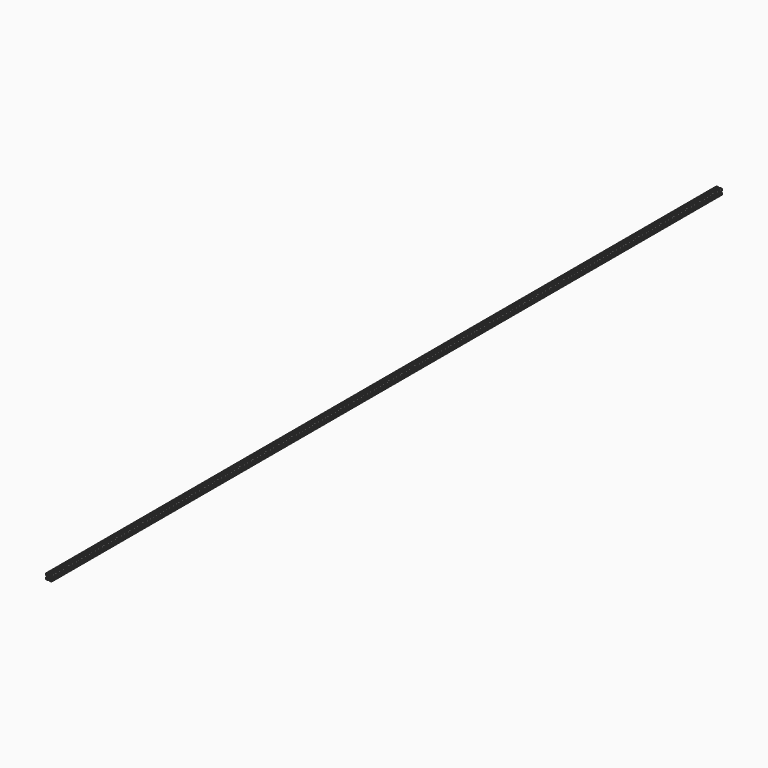
from build123d import *

# Parameters (mm, degrees)
F0_R     = 2.6035
F1_DEPTH = 1828.8


# Not quite as in the source:
# - ends of sketch curves that miss each other by under 0.0002 mm in the source are joined


with BuildPart() as f1:
    # F0 (on Front) → F1 (new body, symmetric)
    with BuildSketch(Plane.XZ):
        with BuildLine():
            ThreePointArc((-120.045226, 66.1162), (-119.5372260057, 65.6082762), (-120.0450736, 65.1002000229))
            ThreePointArc((-120.0450736, 65.1002000229), (-119.4277485161, 63.5840774839), (-117.9116260074, 62.9667530175))
            ThreePointArc((-117.9116260074, 62.9667530175), (-117.4035498, 63.4745999943), (-116.895626, 62.9666))
            Line((-116.895626, 62.9666), (-113.6783096, 62.9666))
            ThreePointArc((-113.6783096, 62.9666), (-113.1703096, 63.4746), (-112.6623096, 62.9666))
            Line((-112.6623096, 62.9666), (-111.688626, 62.9666))
            ThreePointArc((-111.688626, 62.9666), (-110.583726, 64.0715), (-111.688626, 65.1764))
            Line((-111.688626, 65.1764), (-113.8200162, 65.1764))
            ThreePointArc((-113.8200162, 65.1764), (-114.758677805, 65.8035936327), (-114.5384366897, 66.9108204897))
            Line((-114.5384366897, 66.9108204897), (-111.2083882, 70.2408552))
            ThreePointArc((-111.2083882, 70.2408552), (-110.1783528978, 70.9291175157), (-108.963333, 71.1708))
            Line((-108.963333, 71.1708), (-105.727119, 71.1708))
            ThreePointArc((-105.727119, 71.1708), (-104.5120991022, 70.9291175157), (-103.4820549697, 70.2408640303))
            Line((-103.4820549697, 70.2408640303), (-100.1520222, 66.9108136))
            ThreePointArc((-100.1520222, 66.9108136), (-99.931774195, 65.8035936327), (-100.8704358, 65.1764))
            Line((-100.8704358, 65.1764), (-103.001826, 65.1764))
            ThreePointArc((-103.001826, 65.1764), (-104.106726, 64.0715), (-103.001826, 62.9666))
            Line((-103.001826, 62.9666), (-102.0281424, 62.9666))
            ThreePointArc((-102.0281424, 62.9666), (-101.5201424, 63.4746), (-101.0121424, 62.9666))
            Line((-101.0121424, 62.9666), (-97.794826, 62.9666))
            ThreePointArc((-97.794826, 62.9666), (-97.2869022, 63.4745999943), (-96.7788260229, 62.9667524))
            ThreePointArc((-96.7788260229, 62.9667524), (-95.2627034839, 63.5840774839), (-94.6453790175, 65.1001999926))
            ThreePointArc((-94.6453790175, 65.1001999926), (-95.1532259943, 65.6082762), (-94.645226, 66.1162))
            Line((-94.645226, 66.1162), (-94.645226, 69.3335164))
            ThreePointArc((-94.645226, 69.3335164), (-95.153226, 69.8415164), (-94.645226, 70.3495164))
            Line((-94.645226, 70.3495164), (-94.645226, 71.3232))
            ThreePointArc((-94.645226, 71.3232), (-95.750126, 72.4281), (-96.855026, 71.3232))
            Line((-96.855026, 71.3232), (-96.855026, 69.1918098))
            ThreePointArc((-96.855026, 69.1918098), (-97.4822196327, 68.253148195), (-98.5894464897, 68.4733893103))
            Line((-98.5894464897, 68.4733893103), (-101.9194812, 71.8034378))
            ThreePointArc((-101.9194812, 71.8034378), (-102.6077435157, 72.8334731022), (-102.849426, 74.048493))
            Line((-102.849426, 74.048493), (-102.849426, 77.284707))
            ThreePointArc((-102.849426, 77.284707), (-102.6077435157, 78.4997268978), (-101.9194900303, 79.5297710303))
            Line((-101.9194900303, 79.5297710303), (-98.5894396, 82.8598038))
            ThreePointArc((-98.5894396, 82.8598038), (-97.4822196327, 83.080051805), (-96.855026, 82.1413902))
            Line((-96.855026, 82.1413902), (-96.855026, 80.01))
            ThreePointArc((-96.855026, 80.01), (-95.750126, 78.9051), (-94.645226, 80.01))
            Line((-94.645226, 80.01), (-94.645226, 80.9836836))
            ThreePointArc((-94.645226, 80.9836836), (-95.153226, 81.4916836), (-94.645226, 81.9996836))
            Line((-94.645226, 81.9996836), (-94.645226, 85.217))
            ThreePointArc((-94.645226, 85.217), (-95.1532259943, 85.7249238), (-94.6453784, 86.2329999771))
            ThreePointArc((-94.6453784, 86.2329999771), (-95.2627034839, 87.7491225161), (-96.7788259926, 88.3664469825))
            ThreePointArc((-96.7788259926, 88.3664469825), (-97.2869022, 87.8586000057), (-97.794826, 88.3666))
            Line((-97.794826, 88.3666), (-101.0121424, 88.3666))
            ThreePointArc((-101.0121424, 88.3666), (-101.5201424, 87.8586), (-102.0281424, 88.3666))
            Line((-102.0281424, 88.3666), (-103.001826, 88.3666))
            ThreePointArc((-103.001826, 88.3666), (-104.106726, 87.2617), (-103.001826, 86.1568))
            Line((-103.001826, 86.1568), (-100.8704358, 86.1568))
            ThreePointArc((-100.8704358, 86.1568), (-99.931774195, 85.5296063673), (-100.1520153103, 84.4223795103))
            Line((-100.1520153103, 84.4223795103), (-103.4820638, 81.0923448))
            ThreePointArc((-103.4820638, 81.0923448), (-104.5120991022, 80.4040824843), (-105.727119, 80.1624))
            Line((-105.727119, 80.1624), (-108.963333, 80.1624))
            ThreePointArc((-108.963333, 80.1624), (-110.1783528978, 80.4040824843), (-111.2083970303, 81.0923359697))
            Line((-111.2083970303, 81.0923359697), (-114.5384298, 84.4223864))
            ThreePointArc((-114.5384298, 84.4223864), (-114.758677805, 85.5296063673), (-113.8200162, 86.1568))
            Line((-113.8200162, 86.1568), (-111.688626, 86.1568))
            ThreePointArc((-111.688626, 86.1568), (-110.583726, 87.2617), (-111.688626, 88.3666))
            Line((-111.688626, 88.3666), (-112.6623096, 88.3666))
            ThreePointArc((-112.6623096, 88.3666), (-113.1703096, 87.8586), (-113.6783096, 88.3666))
            Line((-113.6783096, 88.3666), (-116.895626, 88.3666))
            ThreePointArc((-116.895626, 88.3666), (-117.4035498, 87.8586000057), (-117.9116259771, 88.3664476))
            ThreePointArc((-117.9116259771, 88.3664476), (-119.4277485161, 87.7491225161), (-120.0450729825, 86.2330000074))
            ThreePointArc((-120.0450729825, 86.2330000074), (-119.5372260057, 85.7249238), (-120.045226, 85.217))
            Line((-120.045226, 85.217), (-120.045226, 81.9996836))
            ThreePointArc((-120.045226, 81.9996836), (-119.537226, 81.4916836), (-120.045226, 80.9836836))
            Line((-120.045226, 80.9836836), (-120.045226, 80.01))
            ThreePointArc((-120.045226, 80.01), (-118.940326, 78.9051), (-117.835426, 80.01))
            Line((-117.835426, 80.01), (-117.835426, 82.1413902))
            ThreePointArc((-117.835426, 82.1413902), (-117.2082323673, 83.080051805), (-116.1010055103, 82.8598106897))
            Line((-116.1010055103, 82.8598106897), (-112.7709708, 79.5297622))
            ThreePointArc((-112.7709708, 79.5297622), (-112.0827084843, 78.4997268978), (-111.841026, 77.284707))
            Line((-111.841026, 77.284707), (-111.841026, 74.048493))
            ThreePointArc((-111.841026, 74.048493), (-112.0827084843, 72.8334731022), (-112.7709619697, 71.8034289697))
            Line((-112.7709619697, 71.8034289697), (-116.1010124, 68.4733962))
            ThreePointArc((-116.1010124, 68.4733962), (-117.2082323673, 68.253148195), (-117.835426, 69.1918098))
            Line((-117.835426, 69.1918098), (-117.835426, 71.3232))
            ThreePointArc((-117.835426, 71.3232), (-118.940326, 72.4281), (-120.045226, 71.3232))
            Line((-120.045226, 71.3232), (-120.045226, 70.3495164))
            ThreePointArc((-120.045226, 70.3495164), (-119.537226, 69.8415164), (-120.045226, 69.3335164))
            Line((-120.045226, 69.3335164), (-120.045226, 66.1162))
        make_face()
        with Locations((-107.345226, 75.6666)):
            Circle(F0_R, mode=Mode.SUBTRACT)
    extrude(amount=F1_DEPTH, both=True)


solid = f1.part
